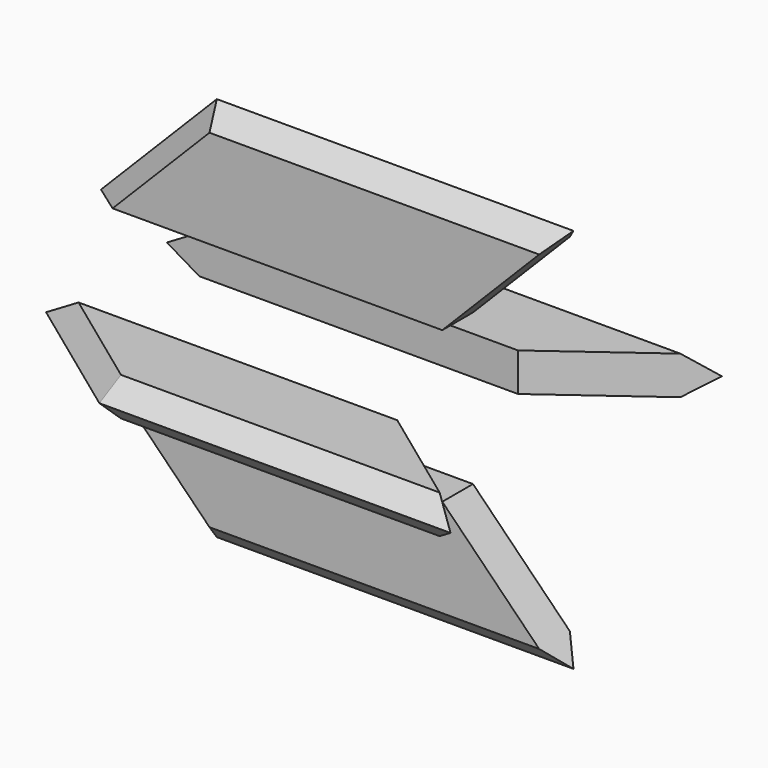
from build123d import *

# Parameters (mm, degrees)
F2_DEPTH      = 2.54
F3_DEPTH      = 2.54
F4_T1_DEPTH   = 76.9282991577
F4_2_T1_DEPTH = 76.9282991577
F4_3_T1_DEPTH = 76.9282991577
F4_4_T1_DEPTH = 76.9282991577
F5_T1_DEPTH   = 44.3887766137
F5_2_T1_DEPTH = 42.9277887493
F5_3_T1_DEPTH = 44.3887766137
F5_4_T1_DEPTH = 42.9277887493


# Not quite as in the source:
# - a fillet or chamfer that OpenCascade refuses, or shapes differently, is made with other operations: its cross-section is extruded or revolved along the edge and cut away or added


with BuildPart() as f2:
    # F0 (on Top) → F2 (new body, symmetric)
    with BuildSketch(Plane.XY):
        Polygon((-25.4, 10), (25.4, 10), (45.8957331301, 25.0028305149), (-4.9042668699, 25.0028305149), align=None)
    extrude(amount=F2_DEPTH, both=True)

    # F4#3: chamfer of 5.08 on 2 edges, made by hand

    # F4_3_s2 → F4_3_t1 (cut)
    with BuildSketch(Plane.YZ.offset(-17.9684164487)):
        Polygon((25.0028305149, -2.54), (19.9228305149, 2.54), (25.0028305149, 2.54), align=None)
        Polygon((25.0028305149, 2.54), (19.9228305149, -2.54), (25.0028305149, -2.54), align=None)
    extrude(amount=F4_3_T1_DEPTH, mode=Mode.SUBTRACT)

    # F5#2: chamfer of 5.08 on 2 edges, made by hand

    # F5_2_s2 → F5_2_t1 (cut)
    with BuildSketch(Plane(origin=(12.3253045755, 9.0220952047, 0), x_dir=(0, 0, 1), z_dir=(-0.8069186272, -0.5906626187, 0))):
        Polygon((-2.54, 17.9920167866), (2.54, 23.0720167866), (-2.54, 23.0720167866), align=None)
        Polygon((-2.54, 23.0720167866), (2.54, 17.9920167866), (2.54, 23.0720167866), align=None)
    extrude(amount=F5_2_T1_DEPTH, mode=Mode.SUBTRACT)


with BuildPart() as f2b:
    # F0 (on Top) → F2, piece 2 (new body, symmetric)
    with BuildSketch(Plane.XY):
        Polygon((45.8957331301, -25.0028305149), (25.4, -10), (-25.4, -10), (-4.9042668699, -25.0028305149), align=None)
    extrude(amount=F2_DEPTH, both=True)

    # F4: chamfer of 5.08 on 2 edges, made by hand

    # F4_s2 → F4_t1 (cut)
    with BuildSketch(Plane.YZ.offset(-17.9684164487)):
        Polygon((-25.0028305149, 2.54), (-19.9228305149, -2.54), (-25.0028305149, -2.54), align=None)
        Polygon((-25.0028305149, -2.54), (-19.9228305149, 2.54), (-25.0028305149, 2.54), align=None)
    extrude(amount=F4_T1_DEPTH, mode=Mode.SUBTRACT)

    # F5#4: chamfer of 5.08 on 2 edges, made by hand

    # F5_4_s2 → F5_4_t1 (cut)
    with BuildSketch(Plane(origin=(-22.3139277895, 16.3337449128, 0), x_dir=(0, 0, 1), z_dir=(0.8069186272, -0.5906626187, 0))):
        Polygon((2.54, 17.9920167866), (-2.54, 23.0720167866), (2.54, 23.0720167866), align=None)
        Polygon((-2.54, 17.9920167866), (2.54, 23.0720167866), (-2.54, 23.0720167866), align=None)
    extrude(amount=F5_4_T1_DEPTH, mode=Mode.SUBTRACT)


with BuildPart() as f3:
    # F1 (on Front) → F3 (new body, symmetric)
    with BuildSketch(Plane.XZ):
        Polygon((-25.4, 10), (25.4, 10), (43.2473993288, 28.0729172299), (-7.5526006712, 28.0729172299), align=None)
    extrude(amount=F3_DEPTH, both=True)

    # F4#2: chamfer of 5.08 on 2 edges, made by hand

    # F4_2_s2 → F4_2_t1 (cut)
    with BuildSketch(Plane.YZ.offset(-20.6167502501)):
        Polygon((-2.54, 28.0729172299), (2.54, 22.9929172299), (2.54, 28.0729172299), align=None)
        Polygon((2.54, 28.0729172299), (-2.54, 22.9929172299), (-2.54, 28.0729172299), align=None)
    extrude(amount=F4_2_T1_DEPTH, mode=Mode.SUBTRACT)

    # F5#3: chamfer of 5.08 on 2 edges, made by hand

    # F5_3_s2 → F5_3_t1 (cut)
    with BuildSketch(Plane(origin=(14.4694272926, 0, 14.6522614868), x_dir=(0, 1, 0), z_dir=(-0.7026535169, 0, -0.7115321744))):
        Polygon((2.54, -20.0194523987), (-2.54, -25.0994523987), (2.54, -25.0994523987), align=None)
        Polygon((2.54, -25.0994523987), (-2.54, -20.0194523987), (-2.54, -25.0994523987), align=None)
    extrude(amount=F5_3_T1_DEPTH, mode=Mode.SUBTRACT)


with BuildPart() as f3b:
    # F1 (on Front) → F3, piece 2 (new body, symmetric)
    with BuildSketch(Plane.XZ):
        Polygon((43.2473993288, -28.0729172299), (25.4, -10), (-25.4, -10), (-7.5526006712, -28.0729172299), align=None)
    extrude(amount=F3_DEPTH, both=True)

    # F4#4: chamfer of 5.08 on 2 edges, made by hand

    # F4_4_s2 → F4_4_t1 (cut)
    with BuildSketch(Plane.YZ.offset(-20.6167502501)):
        Polygon((-2.54, -28.0729172299), (2.54, -22.9929172299), (2.54, -28.0729172299), align=None)
        Polygon((2.54, -28.0729172299), (-2.54, -22.9929172299), (-2.54, -28.0729172299), align=None)
    extrude(amount=F4_4_T1_DEPTH, mode=Mode.SUBTRACT)

    # F5: chamfer of 5.08 on 2 edges, made by hand

    # F5_s2 → F5_t1 (cut)
    with BuildSketch(Plane(origin=(-16.720502705, 0, 16.9317812564), x_dir=(0, 1, 0), z_dir=(0.7026535169, 0, -0.7115321744))):
        Polygon((2.54, -20.0194523987), (-2.54, -25.0994523987), (2.54, -25.0994523987), align=None)
        Polygon((-2.54, -20.0194523987), (2.54, -25.0994523987), (-2.54, -25.0994523987), align=None)
    extrude(amount=F5_T1_DEPTH, mode=Mode.SUBTRACT)


solid = Compound([f2.part, f2b.part, f3.part, f3b.part])
